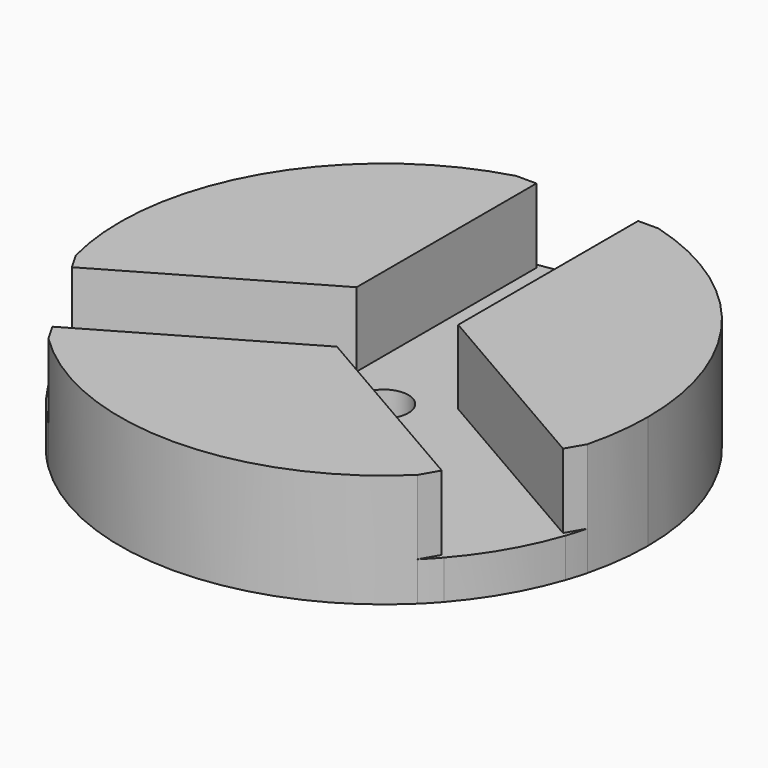
from build123d import *

# Parameters (mm, degrees)
F0_R     = 6.25
F1_DEPTH = 10
F2_DEPTH = 29


# Not quite as in the source:
# - a feature names something its author has since deleted; it is built from what else it names


with BuildPart() as f1:
    # F0 (on Top) → F1 (new body)
    with BuildSketch(Plane.XY):
        with BuildLine():
            Line((13, 65), (18.200275, 65))
            ThreePointArc((18.200275, 65), (15.61238, 65.669655), (13, 66.236319))
            Line((13, 66.236319), (13, 65))
        make_face()
        with BuildLine():
            Line((-13, 65), (-13, 66.236319))
            ThreePointArc((-13, 66.236319), (-15.61238, 65.669655), (-18.200275, 65))
            Line((-18.200275, 65), (-13, 65))
        make_face()
        with BuildLine():
            Line((-62.791651, -21.24167), (-65.391789, -16.7381))
            ThreePointArc((-65.391789, -16.7381), (-64.677779, -19.31411), (-63.862335, -21.859829))
            Line((-63.862335, -21.859829), (-62.791651, -21.24167))
        make_face()
        with BuildLine():
            ThreePointArc((-50.862335, -44.37649), (-49.0654, -46.355545), (-47.191514, -48.2619))
            Line((-47.191514, -48.2619), (-49.791651, -43.75833))
            Line((-49.791651, -43.75833), (-50.862335, -44.37649))
        make_face()
        with BuildLine():
            ThreePointArc((47.191514, -48.2619), (49.0654, -46.355545), (50.862335, -44.37649))
            Line((50.862335, -44.37649), (49.791651, -43.75833))
            Line((49.791651, -43.75833), (47.191514, -48.2619))
        make_face()
        with BuildLine():
            ThreePointArc((63.862335, -21.859829), (64.677779, -19.31411), (65.391789, -16.7381))
            Line((65.391789, -16.7381), (62.791651, -21.24167))
            Line((62.791651, -21.24167), (63.862335, -21.859829))
        make_face()
        with BuildLine():
            Line((-13, 7.505553), (-13, 65))
            Line((-13, 65), (-18.200275, 65))
            ThreePointArc((-18.200275, 65), (-58.456715, 33.75), (-65.391789, -16.7381))
            Line((-65.391789, -16.7381), (-62.791651, -21.24167))
            Line((-62.791651, -21.24167), (-13, 7.505553))
        make_face()
        with BuildLine():
            Line((-49.791651, -43.75833), (-62.791651, -21.24167))
            Line((-62.791651, -21.24167), (-63.862335, -21.859829))
            ThreePointArc((-63.862335, -21.859829), (-58.456715, -33.75), (-50.862335, -44.37649))
            Line((-50.862335, -44.37649), (-49.791651, -43.75833))
        make_face()
        with BuildLine():
            Line((47.191514, -48.2619), (49.791651, -43.75833))
            Line((49.791651, -43.75833), (0, -15.011107))
            Line((0, -15.011107), (-49.791651, -43.75833))
            Line((-49.791651, -43.75833), (-47.191514, -48.2619))
            ThreePointArc((-47.191514, -48.2619), (0, -67.5), (47.191514, -48.2619))
        make_face()
        with BuildLine():
            ThreePointArc((50.862335, -44.37649), (58.456715, -33.75), (63.862335, -21.859829))
            Line((63.862335, -21.859829), (62.791651, -21.24167))
            Line((62.791651, -21.24167), (49.791651, -43.75833))
            Line((49.791651, -43.75833), (50.862335, -44.37649))
        make_face()
        with BuildLine():
            ThreePointArc((65.391789, -16.7381), (66.970873, -8.435172), (67.5, 0))
            ThreePointArc((67.5, 0), (53.780891, 40.79051), (18.200275, 65))
            Line((18.200275, 65), (13, 65))
            Line((13, 65), (13, 7.505553))
            Line((13, 7.505553), (62.791651, -21.24167))
            Line((62.791651, -21.24167), (65.391789, -16.7381))
        make_face()
        with BuildLine():
            Line((13, 7.505553), (13, 65))
            Line((13, 65), (-13, 65))
            Line((-13, 65), (-13, 7.505553))
            Line((-13, 7.505553), (-6.5, 11.25833))
            ThreePointArc((-6.5, 11.25833), (0, 13), (6.5, 11.25833))
            Line((6.5, 11.25833), (13, 7.505553))
        make_face()
        with BuildLine():
            Line((13, 65), (13, 66.236319))
            ThreePointArc((13, 66.236319), (0, 67.5), (-13, 66.236319))
            Line((-13, 66.236319), (-13, 65))
            Line((-13, 65), (13, 65))
        make_face()
        with BuildLine():
            Line((-13, 0), (-13, 7.505553))
            Line((-13, 7.505553), (-62.791651, -21.24167))
            Line((-62.791651, -21.24167), (-49.791651, -43.75833))
            Line((-49.791651, -43.75833), (0, -15.011107))
            Line((0, -15.011107), (-6.5, -11.25833))
            ThreePointArc((-6.5, -11.25833), (-11.25833, -6.5), (-13, 0))
        make_face()
        with BuildLine():
            Line((-6.5, -11.25833), (0, -15.011107))
            Line((0, -15.011107), (6.5, -11.25833))
            ThreePointArc((6.5, -11.25833), (0, -13), (-6.5, -11.25833))
        make_face()
        with BuildLine():
            Line((-6.5, 11.25833), (-13, 7.505553))
            Line((-13, 7.505553), (-13, 0))
            ThreePointArc((-13, 0), (-11.25833, 6.5), (-6.5, 11.25833))
        make_face()
        with BuildLine():
            Line((13, 0), (13, 7.505553))
            Line((13, 7.505553), (6.5, 11.25833))
            ThreePointArc((6.5, 11.25833), (11.25833, 6.5), (13, 0))
        make_face()
        with BuildLine():
            Line((49.791651, -43.75833), (62.791651, -21.24167))
            Line((62.791651, -21.24167), (13, 7.505553))
            Line((13, 7.505553), (13, 0))
            ThreePointArc((13, 0), (11.25833, -6.5), (6.5, -11.25833))
            Line((6.5, -11.25833), (0, -15.011107))
            Line((0, -15.011107), (49.791651, -43.75833))
        make_face()
        with BuildLine():
            ThreePointArc((6.5, -11.25833), (11.25833, -6.5), (13, 0))
            ThreePointArc((13, 0), (11.25833, 6.5), (6.5, 11.25833))
            ThreePointArc((6.5, 11.25833), (0, 13), (-6.5, 11.25833))
            ThreePointArc((-6.5, 11.25833), (-11.25833, 6.5), (-13, 0))
            ThreePointArc((-13, 0), (-11.25833, -6.5), (-6.5, -11.25833))
            ThreePointArc((-6.5, -11.25833), (0, -13), (6.5, -11.25833))
        make_face()
        Circle(F0_R, mode=Mode.SUBTRACT)
    extrude(amount=F1_DEPTH)

    # F0 (on Top) → F2 (join)
    with BuildSketch(Plane.XY):
        with BuildLine():
            Line((-13, 7.505553), (-13, 65))
            Line((-13, 65), (-18.200275, 65))
            ThreePointArc((-18.200275, 65), (-58.456715, 33.75), (-65.391789, -16.7381))
            Line((-65.391789, -16.7381), (-62.791651, -21.24167))
            Line((-62.791651, -21.24167), (-13, 7.505553))
        make_face()
        with BuildLine():
            Line((47.191514, -48.2619), (49.791651, -43.75833))
            Line((49.791651, -43.75833), (0, -15.011107))
            Line((0, -15.011107), (-49.791651, -43.75833))
            Line((-49.791651, -43.75833), (-47.191514, -48.2619))
            ThreePointArc((-47.191514, -48.2619), (0, -67.5), (47.191514, -48.2619))
        make_face()
        with BuildLine():
            ThreePointArc((65.391789, -16.7381), (66.970873, -8.435172), (67.5, 0))
            ThreePointArc((67.5, 0), (53.780891, 40.79051), (18.200275, 65))
            Line((18.200275, 65), (13, 65))
            Line((13, 65), (13, 7.505553))
            Line((13, 7.505553), (62.791651, -21.24167))
            Line((62.791651, -21.24167), (65.391789, -16.7381))
        make_face()
    extrude(amount=F2_DEPTH)


solid = f1.part
